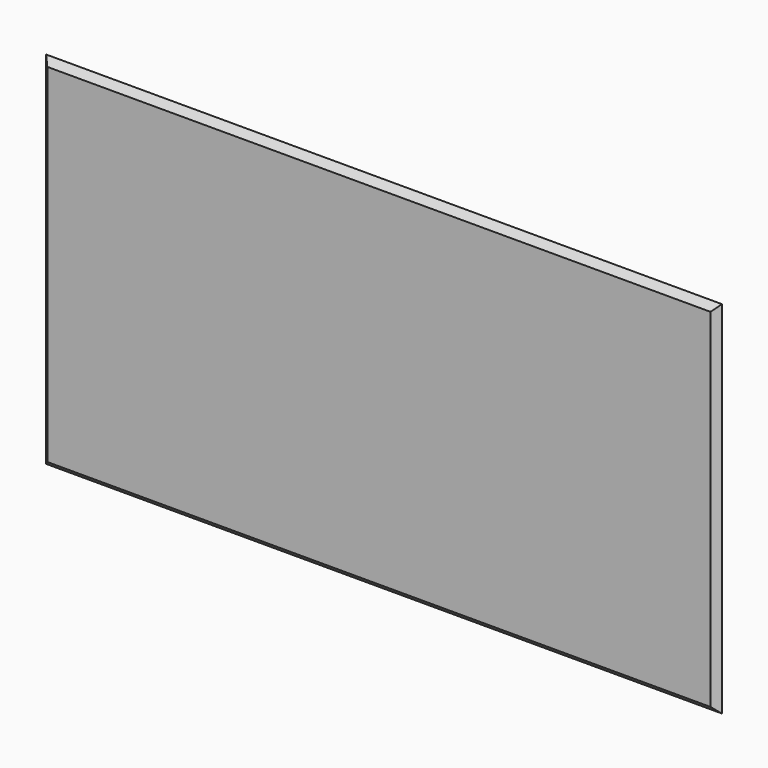
from build123d import *

# Parameters (mm, degrees)
F0_W     = 1500
F0_H     = 800
F1_DEPTH = 14
F2_SIZE  = 13.99999


# Not quite as in the source:
# - a fillet or chamfer is up to 0.001 mm smaller than in the source, because OpenCascade refuses the exact size


with BuildPart() as f1:
    # F0 (on Front) → F1 (new body)
    with BuildSketch(Plane.XZ):
        Rectangle(F0_W, F0_H)
    extrude(amount=F1_DEPTH)

    # F2 (size 14 in the source; OpenCascade refuses exactly that, so slightly less here)
    f2_edges = [f1.edges().sort_by_distance(p)[0] for p in [
        (750, -14, 0),
        (0, -14, 400),
        (-750, -14, 0),
        (0, -14, -400),
    ]]
    chamfer(f2_edges, length=F2_SIZE)


solid = f1.part
